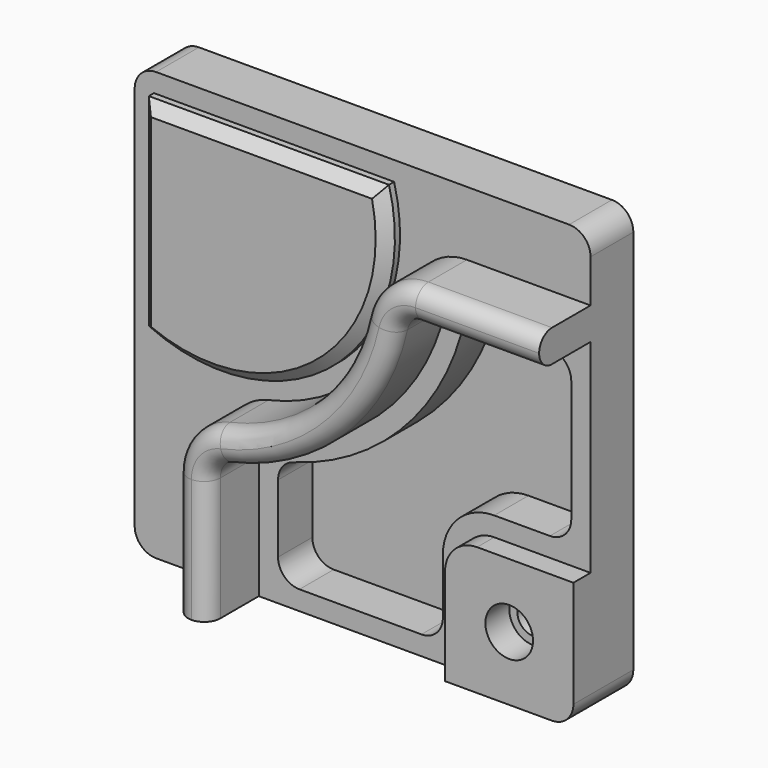
from build123d import *

# Parameters (mm, degrees)
F1_DEPTH       = 25
F2_DEPTH       = 10
F3_DEPTH       = 30
F4_DEPTH       = 20
F5_DEPTH       = 8
F6_SIZE2       = 5
F6_SIZE        = 5
F8_D           = 14.75
F8_CBORE_D     = 22.25
F8_CBORE_DEPTH = 14
F9_R           = 7.49999


# Not quite as in the source:
# - a fillet or chamfer is up to 0.001 mm smaller than in the source, because OpenCascade refuses the exact size


with BuildPart() as f1:
    # F0 (on Front) → F1 (new body)
    with BuildSketch(Plane.XZ):
        with BuildLine():
            Line((106.5, -40), (106.5, 55))
            Line((106.5, 55), (48.7497216032, 55))
            ThreePointArc((48.7497216032, 55), (42.4942891815, 52.8018949761), (38.9888762464, 47.1739130435))
            ThreePointArc((38.9888762464, 47.1739130435), (10.7462120246, -4.2462120246), (-40.6739130435, -32.4888762464))
            ThreePointArc((-40.6739130435, -32.4888762464), (-46.3018949761, -35.9942891815), (-48.5, -42.2497216032))
            Line((-48.5, -42.2497216032), (-48.5, -100))
            Line((-48.5, -100), (46.5, -100))
            Line((46.5, -100), (46.5, -55))
            ThreePointArc((46.5, -55), (50.8933982822, -44.3933982822), (61.5, -40))
            Line((61.5, -40), (106.5, -40))
        make_face()
        with BuildLine():
            ThreePointArc((-29.5, -91), (-36.5710678119, -88.0710678119), (-39.5, -81))
            Line((-39.5, -81), (-39.5, -49.2476414861))
            ThreePointArc((-39.5, -49.2476414861), (-37.481834214, -43.2234965193), (-32.2419354839, -39.630896205))
            ThreePointArc((-32.2419354839, -39.630896205), (17.1101730553, -10.6101730553), (46.130896205, 38.7419354839))
            ThreePointArc((46.130896205, 38.7419354839), (49.7234965193, 43.981834214), (55.7476414861, 46))
            Line((55.7476414861, 46), (87.5, 46))
            ThreePointArc((87.5, 46), (94.5710678119, 43.0710678119), (97.5, 36))
            Line((97.5, 36), (97.5, -21))
            ThreePointArc((97.5, -21), (94.5710678119, -28.0710678119), (87.5, -31))
            Line((87.5, -31), (61.5, -31))
            ThreePointArc((61.5, -31), (44.5294372515, -38.0294372515), (37.5, -55))
            Line((37.5, -55), (37.5, -81))
            ThreePointArc((37.5, -81), (34.5710678119, -88.0710678119), (27.5, -91))
            Line((27.5, -91), (-29.5, -91))
        make_face(mode=Mode.SUBTRACT)
        with BuildLine():
            Line((96.5, 100), (-96.5, 100))
            ThreePointArc((-96.5, 100), (-103.5710678119, 97.0710678119), (-106.5, 90))
            Line((-106.5, 90), (-106.5, -90))
            ThreePointArc((-106.5, -90), (-103.5710678119, -97.0710678119), (-96.5, -100))
            Line((-96.5, -100), (-63.5, -100))
            Line((-63.5, -100), (-63.5, -42.2497216032))
            ThreePointArc((-63.5, -42.2497216032), (-58.0047374401, -26.6111405489), (-43.9347826087, -17.8476082112))
            ThreePointArc((-43.9347826087, -17.8476082112), (0.1396103068, 6.3603896932), (24.3476082112, 50.4347826087))
            ThreePointArc((24.3476082112, 50.4347826087), (33.1111405489, 64.5047374401), (48.7497216032, 70))
            Line((48.7497216032, 70), (106.5, 70))
            Line((106.5, 70), (106.5, 90))
            ThreePointArc((106.5, 90), (103.5710678119, 97.0710678119), (96.5, 100))
        make_face()
        with BuildLine():
            ThreePointArc((14.7304288624, 91), (-11.3221396288, 8.044605666), (-97.5, -3.5187051029))
            Line((-97.5, -3.5187051029), (-97.5, 91))
            Line((-97.5, 91), (14.7304288624, 91))
        make_face(mode=Mode.SUBTRACT)
        with BuildLine():
            Line((-97.5, 91), (-97.5, -3.5187051029))
            ThreePointArc((-97.5, -3.5187051029), (-11.3221396288, 8.044605666), (14.7304288624, 91))
            Line((14.7304288624, 91), (-97.5, 91))
        make_face()
        with BuildLine():
            Line((-39.5, -49.2476414861), (-39.5, -81))
            ThreePointArc((-39.5, -81), (-36.5710678119, -88.0710678119), (-29.5, -91))
            Line((-29.5, -91), (27.5, -91))
            ThreePointArc((27.5, -91), (34.5710678119, -88.0710678119), (37.5, -81))
            Line((37.5, -81), (37.5, -55))
            ThreePointArc((37.5, -55), (44.5294372515, -38.0294372515), (61.5, -31))
            Line((61.5, -31), (87.5, -31))
            ThreePointArc((87.5, -31), (94.5710678119, -28.0710678119), (97.5, -21))
            Line((97.5, -21), (97.5, 36))
            ThreePointArc((97.5, 36), (94.5710678119, 43.0710678119), (87.5, 46))
            Line((87.5, 46), (55.7476414861, 46))
            ThreePointArc((55.7476414861, 46), (49.7234965193, 43.981834214), (46.130896205, 38.7419354839))
            ThreePointArc((46.130896205, 38.7419354839), (17.1101730553, -10.6101730553), (-32.2419354839, -39.630896205))
            ThreePointArc((-32.2419354839, -39.630896205), (-37.481834214, -43.2234965193), (-39.5, -49.2476414861))
        make_face()
        with BuildLine():
            Line((106.5, 55), (106.5, 70))
            Line((106.5, 70), (48.7497216032, 70))
            ThreePointArc((48.7497216032, 70), (33.1111405489, 64.5047374401), (24.3476082112, 50.4347826087))
            ThreePointArc((24.3476082112, 50.4347826087), (0.1396103068, 6.3603896932), (-43.9347826087, -17.8476082112))
            ThreePointArc((-43.9347826087, -17.8476082112), (-58.0047374401, -26.6111405489), (-63.5, -42.2497216032))
            Line((-63.5, -42.2497216032), (-63.5, -100))
            Line((-63.5, -100), (-48.5, -100))
            Line((-48.5, -100), (-48.5, -42.2497216032))
            ThreePointArc((-48.5, -42.2497216032), (-46.3018949761, -35.9942891815), (-40.6739130435, -32.4888762464))
            ThreePointArc((-40.6739130435, -32.4888762464), (10.7462120246, -4.2462120246), (38.9888762464, 47.1739130435))
            ThreePointArc((38.9888762464, 47.1739130435), (42.4942891815, 52.8018949761), (48.7497216032, 55))
            Line((48.7497216032, 55), (106.5, 55))
        make_face()
        with BuildLine():
            Line((106.5, -90), (106.5, -40))
            Line((106.5, -40), (61.5, -40))
            ThreePointArc((61.5, -40), (50.8933982822, -44.3933982822), (46.5, -55))
            Line((46.5, -55), (46.5, -100))
            Line((46.5, -100), (96.5, -100))
            ThreePointArc((96.5, -100), (103.5710678119, -97.0710678119), (106.5, -90))
        make_face()
    extrude(amount=-F1_DEPTH)

    # F0 (on Front) → F2 (join)
    with BuildSketch(Plane.XZ):
        with BuildLine():
            Line((106.5, -90), (106.5, -40))
            Line((106.5, -40), (61.5, -40))
            ThreePointArc((61.5, -40), (50.8933982822, -44.3933982822), (46.5, -55))
            Line((46.5, -55), (46.5, -100))
            Line((46.5, -100), (96.5, -100))
            ThreePointArc((96.5, -100), (103.5710678119, -97.0710678119), (106.5, -90))
        make_face()
    extrude(amount=F2_DEPTH)

    # F0 (on Front) → F3 (join)
    with BuildSketch(Plane.XZ):
        with BuildLine():
            Line((106.5, 55), (106.5, 70))
            Line((106.5, 70), (48.7497216032, 70))
            ThreePointArc((48.7497216032, 70), (33.1111405489, 64.5047374401), (24.3476082112, 50.4347826087))
            ThreePointArc((24.3476082112, 50.4347826087), (0.1396103068, 6.3603896932), (-43.9347826087, -17.8476082112))
            ThreePointArc((-43.9347826087, -17.8476082112), (-58.0047374401, -26.6111405489), (-63.5, -42.2497216032))
            Line((-63.5, -42.2497216032), (-63.5, -100))
            Line((-63.5, -100), (-48.5, -100))
            Line((-48.5, -100), (-48.5, -42.2497216032))
            ThreePointArc((-48.5, -42.2497216032), (-46.3018949761, -35.9942891815), (-40.6739130435, -32.4888762464))
            ThreePointArc((-40.6739130435, -32.4888762464), (10.7462120246, -4.2462120246), (38.9888762464, 47.1739130435))
            ThreePointArc((38.9888762464, 47.1739130435), (42.4942891815, 52.8018949761), (48.7497216032, 55))
            Line((48.7497216032, 55), (106.5, 55))
        make_face()
    extrude(amount=F3_DEPTH)

    # F0 (on Front) → F4 (cut)
    with BuildSketch(Plane.XZ):
        with BuildLine():
            Line((-39.5, -49.2476414861), (-39.5, -81))
            ThreePointArc((-39.5, -81), (-36.5710678119, -88.0710678119), (-29.5, -91))
            Line((-29.5, -91), (27.5, -91))
            ThreePointArc((27.5, -91), (34.5710678119, -88.0710678119), (37.5, -81))
            Line((37.5, -81), (37.5, -55))
            ThreePointArc((37.5, -55), (44.5294372515, -38.0294372515), (61.5, -31))
            Line((61.5, -31), (87.5, -31))
            ThreePointArc((87.5, -31), (94.5710678119, -28.0710678119), (97.5, -21))
            Line((97.5, -21), (97.5, 36))
            ThreePointArc((97.5, 36), (94.5710678119, 43.0710678119), (87.5, 46))
            Line((87.5, 46), (55.7476414861, 46))
            ThreePointArc((55.7476414861, 46), (49.7234965193, 43.981834214), (46.130896205, 38.7419354839))
            ThreePointArc((46.130896205, 38.7419354839), (17.1101730553, -10.6101730553), (-32.2419354839, -39.630896205))
            ThreePointArc((-32.2419354839, -39.630896205), (-37.481834214, -43.2234965193), (-39.5, -49.2476414861))
        make_face()
    extrude(amount=-F4_DEPTH, mode=Mode.SUBTRACT)

    # F0 (on Front) → F5 (join)
    with BuildSketch(Plane.XZ):
        with BuildLine():
            Line((-97.5, 91), (-97.5, -3.5187051029))
            ThreePointArc((-97.5, -3.5187051029), (-11.3221396288, 8.044605666), (14.7304288624, 91))
            Line((14.7304288624, 91), (-97.5, 91))
        make_face()
    extrude(amount=F5_DEPTH)

    # F6
    f6_edges = [f1.edges().sort_by_distance(p)[0] for p in [
        (-41.384786, -8, 91),
        (-97.5, -8, 43.740647),
        (-11.32214, -8, 8.044606),
    ]]
    chamfer(f6_edges, length=F6_SIZE, length2=F6_SIZE2)

    # F8 (through all)
    with Locations(Plane.XZ.offset(10)):
        with Locations((76.5, -70)):
            CounterBoreHole(F8_D / 2, F8_CBORE_D / 2, F8_CBORE_DEPTH)

    # F9 (radius 7.5 in the source; OpenCascade refuses exactly that, so slightly less here)
    f9_edges = [f1.edges().sort_by_distance(p)[0] for p in [
        (-48.5, -30, -71.124861),
        (-63.5, -30, -71.124861),
    ]]
    fillet(f9_edges, radius=F9_R)


solid = f1.part
